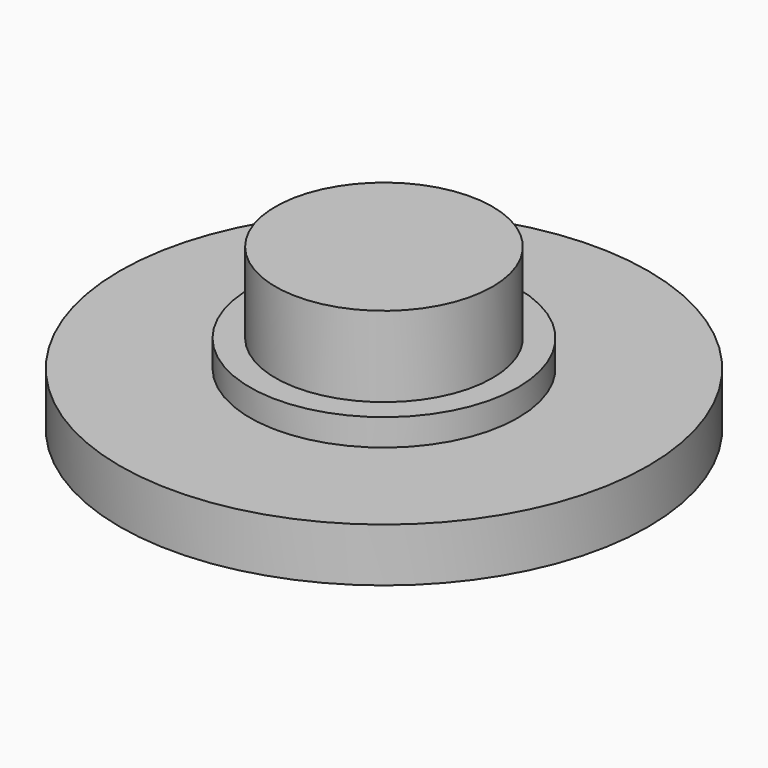
from build123d import *

# Parameters (mm, degrees)
F0_R     = 9.8592181747
F1_DEPTH = 2
F2_R     = 5
F3_DEPTH = 1
F4_R     = 4.05
F5_DEPTH = 3
F6_R     = 8.2811029309
F7_DEPTH = 1


# Not quite as in the source:
# - a fillet or chamfer that OpenCascade refuses, or shapes differently, is made with other operations: its cross-section is extruded or revolved along the edge and cut away or added


with BuildPart() as f1:
    # F0 (on Top) → F1 (new body)
    with BuildSketch(Plane.XY):
        Circle(F0_R)
    extrude(amount=F1_DEPTH)

    # F2 (on face) → F3 (join)
    with BuildSketch(Plane.XY.offset(2)):
        Circle(F2_R)
    extrude(amount=F3_DEPTH)

    # F4 (on face) → F5 (join)
    with BuildSketch(Plane.XY.offset(3)):
        Circle(F4_R)
    extrude(amount=F5_DEPTH)

    # F6 (on face) → F7 (cut)
    with BuildSketch(Plane(origin=(0, 0, 0), x_dir=(1, 0, 0), z_dir=(0, 0, -1))):
        Circle(F6_R)
    extrude(amount=-F7_DEPTH, mode=Mode.SUBTRACT)

    # F8: fillet of radius 32 on 1 edges, made by hand

    # F8_s1 → F8_t2 (revolve)
    with BuildSketch(Plane.XZ):
        with BuildLine():
            ThreePointArc((8.2811029309, 0), (4.3438489977, 0.7490157328), (0.3438489977, 1))
            Line((0.3438489977, 1), (8.2811029309, 1))
            Line((8.2811029309, 1), (8.2811029309, 0))
        make_face()
    revolve(axis=Axis((0, 0, 1), (0, 0, -1)))


solid = f1.part
